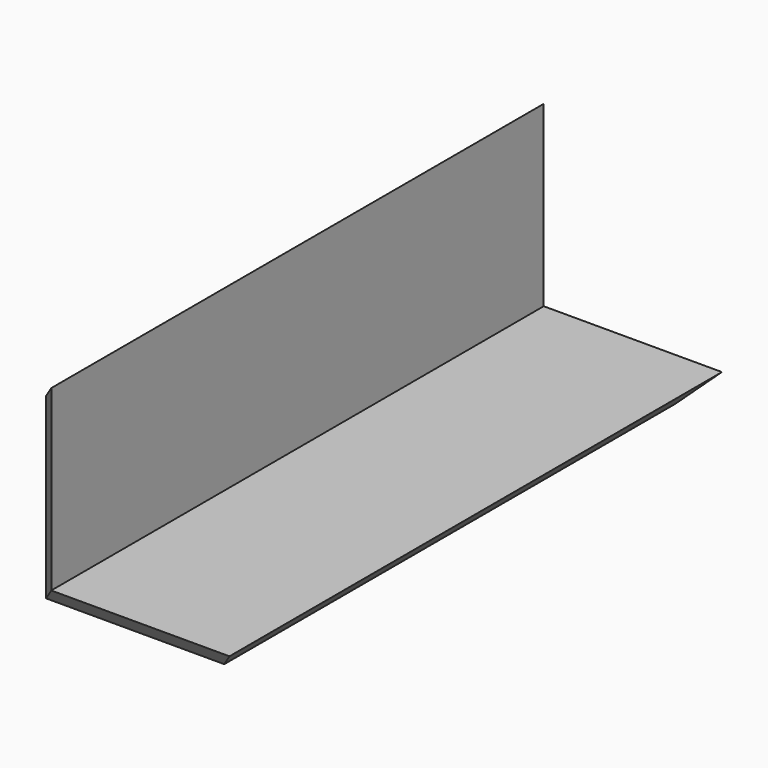
from build123d import *

# Parameters (mm, degrees)
F1_DEPTH = 38
F2_SIZE  = 1.59999


# Not quite as in the source:
# - a fillet or chamfer is up to 0.001 mm smaller than in the source, because OpenCascade refuses the exact size


with BuildPart() as f1:
    # F0 (on Front) → F1 (new body)
    with BuildSketch(Plane.XZ):
        Polygon((0, 12.6), (0, 0), (12.6, 0), (12.6, 1.6), (1.6, 1.6), (1.6, 12.6), align=None)
    extrude(amount=F1_DEPTH)

    # F2 (size 1.6 in the source; OpenCascade refuses exactly that, so slightly less here)
    f2_edges = [f1.edges().sort_by_distance(p)[0] for p in [
        (12.6, -19, 0),
        (0, -19, 12.6),
        (0, 0, 6.3),
        (6.3, 0, 0),
        (0, -38, 6.3),
        (6.3, -38, 0),
    ]]
    chamfer(f2_edges, length=F2_SIZE)


solid = f1.part
